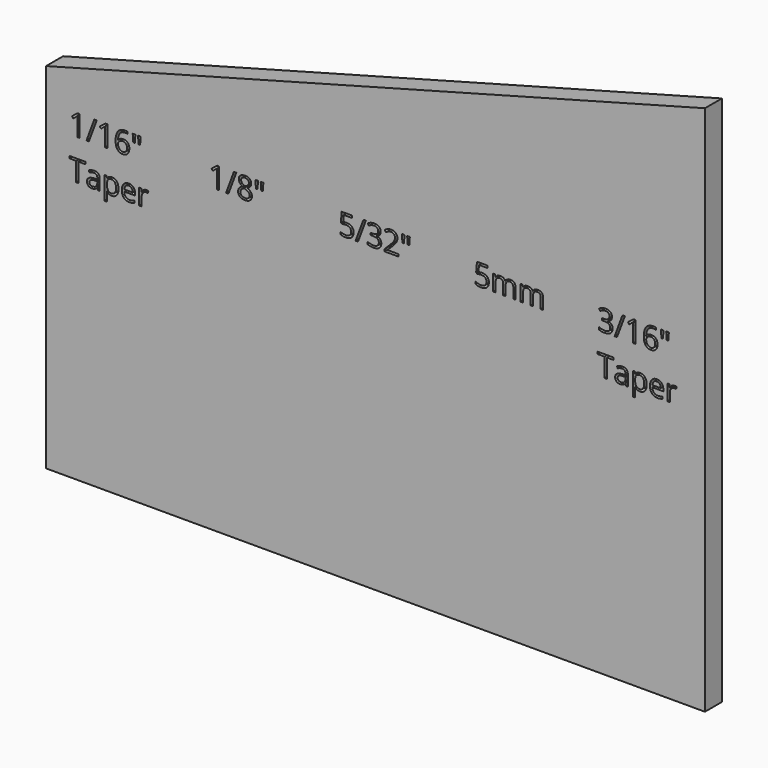
from build123d import *

# Parameters (mm, degrees)
F1_DEPTH     = 3
F2_TEXT_SIZE = 4.1666666667
F3_DEPTH     = 1


# Not quite as in the source:
# - Text() gives the source's letters only with a copy of the font that has no kerning and outlines rounded to 1/6400 em; it was checked with that copy


with BuildPart() as f1:
    # F0 (on Front) → F1 (new body)
    with BuildSketch(Plane.XZ):
        Polygon((0, 50), (0, 0), (93, 0), (93, 75), align=None)
    extrude(amount=-F1_DEPTH)

    # F2 (on Front) → F3 (cut)
    with BuildSketch(Plane.XZ):
        with Locations((3.2797100179, 42.601171899)):
            Text('1/16"', F2_TEXT_SIZE, font='Open Sans', text_align=(TextAlign.LEFT, TextAlign.BOTTOM))
        with Locations((3.2797100179, 36.9345052324)):
            Text('Taper', F2_TEXT_SIZE, font='Open Sans', text_align=(TextAlign.LEFT, TextAlign.BOTTOM))
        with Locations((22.977925837, 42.4960465431)):
            Text('1/8"', F2_TEXT_SIZE, font='Open Sans', text_align=(TextAlign.LEFT, TextAlign.BOTTOM))
        with Locations((41.2701778114, 42.4960465431)):
            Text('5/32"', F2_TEXT_SIZE, font='Open Sans', text_align=(TextAlign.LEFT, TextAlign.BOTTOM))
        with Locations((60.3664889932, 42.4960502684)):
            Text('5mm', F2_TEXT_SIZE, font='Open Sans', text_align=(TextAlign.LEFT, TextAlign.BOTTOM))
        with Locations((77.8341367841, 42.5228947103)):
            Text('3/16"', F2_TEXT_SIZE, font='Open Sans', text_align=(TextAlign.LEFT, TextAlign.BOTTOM))
        with Locations((77.8341367841, 36.8562280436)):
            Text('Taper', F2_TEXT_SIZE, font='Open Sans', text_align=(TextAlign.LEFT, TextAlign.BOTTOM))
    extrude(amount=-F3_DEPTH, mode=Mode.SUBTRACT)


solid = f1.part
